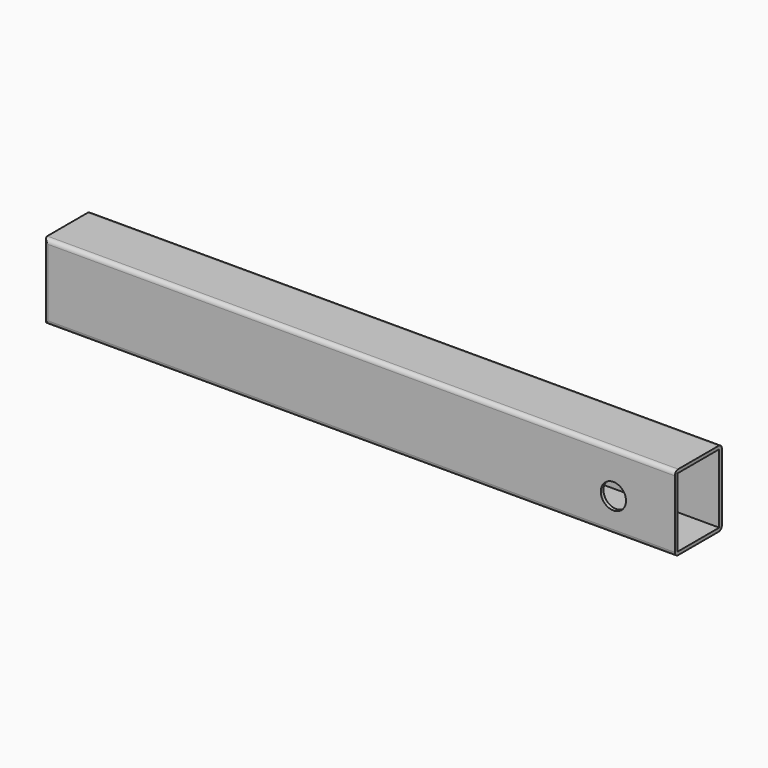
from build123d import *

# Parameters (mm, degrees)
F1_DEPTH     = 70
F2_T         = 4
F3_T1_DEPTH  = 774.9998275448
F3_T3_DEPTH  = 114.9996550895
F3_T6_ANGLE  = 90.0000000944
F3_T8_ANGLE  = 89.9999999363
F3_T10_ANGLE = 90.0000000944
F3_T12_ANGLE = 89.9999999363
F4_R         = 15
F5_DEPTH     = 70.001


# Not quite as in the source:
# - a fillet or chamfer that OpenCascade refuses, or shapes differently, is made with other operations: its cross-section is extruded or revolved along the edge and cut away or added
# - a shell that OpenCascade refuses in one call is made with other operations: the cavity is built on its own and cut out


with BuildPart() as f1:
    # F0 (on Front) → F1 (new body)
    with BuildSketch(Plane.XZ):
        with BuildLine():
            Line((-374.9998275448, -45), (375, -45))
            Line((375, -45), (375, 45))
            Line((375, 45), (-374.9998275448, 45))
            ThreePointArc((-374.9998275448, 45), (-374.999949489, 44.999949489), (-375, 44.9998275448))
            Line((-375, 44.9998275448), (-375, -44.9998275448))
            ThreePointArc((-375, -44.9998275448), (-374.999949489, -44.999949489), (-374.9998275448, -45))
        make_face()
    extrude(amount=F1_DEPTH)

    # F2: shell of thickness 4, made by hand


with BuildPart() as f2_core1:
    # F2_t2: copy of F1
    add(f1.part)

    # the walls: a layer under each face that stays
    f2_faces = [f2_core1.faces().sort_by_distance(p)[0] for p in [
        (8.62276e-05, -35, -45),
        (8.62276e-05, -35, 45),
        (0, 0, 0),
        (0, -70, 0),
    ]]
    thicken(f2_faces, amount=-F2_T, mode=Mode.SUBTRACT)


with BuildPart() as f1_1:
    add(f1.part)

    # what is left inside the walls is the cavity
    f2_cavity = [f2_core1.part.solids().sort_by_distance(p)[0] for p in [
        (0, -4.04, -15),
    ]]
    add(f2_cavity, mode=Mode.SUBTRACT)

    # F3: fillet of radius 5 on 4 edges, made by hand

    # F3_s2 → F3_t1 (cut)
    with BuildSketch(Plane.YZ.offset(-387.4998275448)):
        with BuildLine():
            ThreePointArc((-70, 40), (-68.5355339059, 43.5355339059), (-65, 45))
            Line((-65, 45), (-70, 45))
            Line((-70, 45), (-70, 40))
        make_face()
        with BuildLine():
            ThreePointArc((0, 40), (-1.4644660941, 43.5355339059), (-5, 45))
            Line((-5, 45), (0, 45))
            Line((0, 45), (0, 40))
        make_face()
        with BuildLine():
            ThreePointArc((-5, -45), (-1.4644660941, -43.5355339059), (0, -40))
            Line((0, -40), (0, -45))
            Line((0, -45), (-5, -45))
        make_face()
        with BuildLine():
            ThreePointArc((-65, -45), (-68.5355339059, -43.5355339059), (-70, -40))
            Line((-70, -40), (-70, -45))
            Line((-70, -45), (-65, -45))
        make_face()
    extrude(amount=F3_T1_DEPTH, mode=Mode.SUBTRACT)

    # F3_s4 → F3_t3 (cut)
    with BuildSketch(Plane.XY.offset(-57.4998275448)):
        with BuildLine():
            ThreePointArc((-370, -70), (-373.5355339059, -68.5355339059), (-375, -65))
            Line((-375, -65), (-375, -70))
            Line((-375, -70), (-370, -70))
        make_face()
        with BuildLine():
            ThreePointArc((-370, 0), (-373.5355339059, -1.4644660941), (-375, -5))
            Line((-375, -5), (-375, 0))
            Line((-375, 0), (-370, 0))
        make_face()
    extrude(amount=F3_T3_DEPTH, mode=Mode.SUBTRACT)

    # F3_s5 → F3_t6 (revolve, cut)
    with BuildSketch(Plane.XY.offset(-44.9998275448)):
        with BuildLine():
            ThreePointArc((-375, -65), (-374.999956886, -65.0207638646), (-374.9998275448, -65.0415273711))
            Line((-374.9998275448, -65.0415273711), (-374.9998275448, -70))
            Line((-374.9998275448, -70), (-375, -70))
            Line((-375, -70), (-375, -65))
        make_face()
    revolve(axis=Axis((-374.9998275448, -70, -44.9998275448), (0, -1, 0)), revolution_arc=F3_T6_ANGLE, mode=Mode.SUBTRACT)

    # F3_s7 → F3_t8 (revolve, cut)
    with BuildSketch(Plane.YZ.offset(-374.9998275448)):
        with BuildLine():
            ThreePointArc((-65.0415273711, 44.9998275448), (-65.0207638646, 44.999956886), (-65, 45))
            Line((-65, 45), (-70, 45))
            Line((-70, 45), (-70, 44.9998275448))
            Line((-70, 44.9998275448), (-65.0415273711, 44.9998275448))
        make_face()
    revolve(axis=Axis((-374.9998275448, -70, 44.9998275448), (0, -1, 0)), revolution_arc=F3_T8_ANGLE, mode=Mode.SUBTRACT)

    # F3_s9 → F3_t10 (revolve, cut)
    with BuildSketch(Plane.XY.offset(-44.9998275448)):
        with BuildLine():
            ThreePointArc((-375, -5), (-374.999956886, -4.9792361354), (-374.9998275448, -4.9584726289))
            Line((-374.9998275448, -4.9584726289), (-374.9998275448, 0))
            Line((-374.9998275448, 0), (-375, 0))
            Line((-375, 0), (-375, -5))
        make_face()
    revolve(axis=Axis((-374.9998275448, 0, -44.9998275448), (0, -1, 0)), revolution_arc=F3_T10_ANGLE, mode=Mode.SUBTRACT)

    # F3_s11 → F3_t12 (revolve, cut)
    with BuildSketch(Plane.YZ.offset(-374.9998275448)):
        with BuildLine():
            ThreePointArc((-4.9584726289, 44.9998275448), (-4.9792361354, 44.999956886), (-5, 45))
            Line((-5, 45), (0, 45))
            Line((0, 45), (0, 44.9998275448))
            Line((0, 44.9998275448), (-4.9584726289, 44.9998275448))
        make_face()
    revolve(axis=Axis((-374.9998275448, 0, 44.9998275448), (0, -1, 0)), revolution_arc=F3_T12_ANGLE, mode=Mode.SUBTRACT)

    # F4 (on Front) → F5 (cut, through all)
    with BuildSketch(Plane.XZ):
        with Locations((302, -5)):
            Circle(F4_R)
    extrude(amount=F5_DEPTH, mode=Mode.SUBTRACT)


solid = f1_1.part
